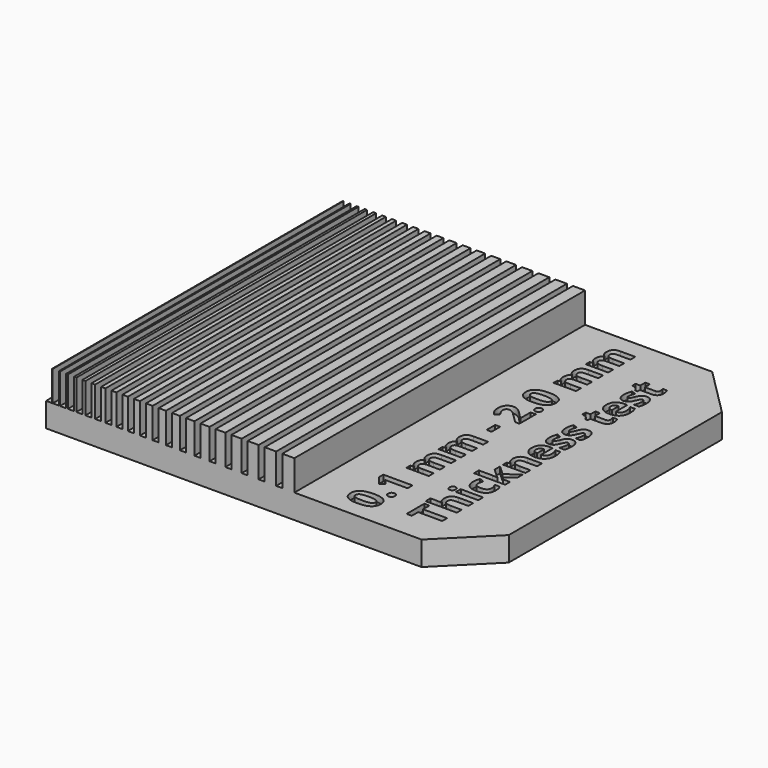
from build123d import *

# Parameters (mm, degrees)
F0_W         = 70
F0_H         = 60
F1_DEPTH     = 4
F2_W         = 0.1
F2_H         = 60
F2_W_2       = 0.2
F2_W_3       = 0.3
F2_W_4       = 0.4
F2_W_5       = 0.5
F2_W_6       = 0.6
F2_W_7       = 0.7
F2_W_8       = 0.8
F2_W_9       = 0.9
F2_W_10      = 1
F2_W_11      = 1.1
F2_W_12      = 1.2
F2_W_13      = 1.3
F2_W_14      = 1.4
F2_W_15      = 1.5
F2_W_16      = 1.6
F2_W_17      = 1.7
F2_W_18      = 1.9
F2_W_19      = 2
F2_W_20      = 1.8
F3_DEPTH     = 5
F4_TEXT_SIZE = 6.7632478961
F5_DEPTH     = 1
F6_SIZE      = 8


# Not quite as in the source:
# - Text() gives the source's letters only with a copy of the font that has no kerning and outlines rounded to 1/6400 em; it was checked with that copy


with BuildPart() as f1:
    # F0 (on Top) → F1 (new body)
    with BuildSketch(Plane.XY):
        Rectangle(F0_W, F0_H)
    extrude(amount=F1_DEPTH)

    # F2 (on face) → F3 (join)
    with BuildSketch(Plane.XY.offset(4)):
        with Locations((-33.95, 0)):
            Rectangle(F2_W, F2_H)
        with Locations((-32.8, 0)):
            Rectangle(F2_W_2, F2_H)
        with Locations((-31.55, 0)):
            Rectangle(F2_W_3, F2_H)
        with Locations((-30.2, 0)):
            Rectangle(F2_W_4, F2_H)
        with Locations((-28.75, 0)):
            Rectangle(F2_W_5, F2_H)
        with Locations((-27.2, 0)):
            Rectangle(F2_W_6, F2_H)
        with Locations((-25.55, 0)):
            Rectangle(F2_W_7, F2_H)
        with Locations((-23.8, 0)):
            Rectangle(F2_W_8, F2_H)
        with Locations((-21.95, 0)):
            Rectangle(F2_W_9, F2_H)
        with Locations((-20, 0)):
            Rectangle(F2_W_10, F2_H)
        with Locations((-17.95, 0)):
            Rectangle(F2_W_11, F2_H)
        with Locations((-15.8, 0)):
            Rectangle(F2_W_12, F2_H)
        with Locations((-13.55, 0)):
            Rectangle(F2_W_13, F2_H)
        with Locations((-11.2, 0)):
            Rectangle(F2_W_14, F2_H)
        with Locations((-8.75, 0)):
            Rectangle(F2_W_15, F2_H)
        with Locations((-6.2, 0)):
            Rectangle(F2_W_16, F2_H)
        with Locations((-3.55, 0)):
            Rectangle(F2_W_17, F2_H)
        with Locations((2.05, 0)):
            Rectangle(F2_W_18, F2_H)
        with Locations((5, 0)):
            Rectangle(F2_W_19, F2_H)
        with Locations((-0.8, 0)):
            Rectangle(F2_W_20, F2_H)
    extrude(amount=F3_DEPTH)

    # F4 (on face) → F5 (cut)
    with BuildSketch(Plane.XY.offset(4)):
        with Locations(Location((16.6463407394, -27.5), (0, 0, 90))):
            Text('0.1 mm - 2.0 mm', F4_TEXT_SIZE, font='Open Sans', font_style=FontStyle.BOLD, text_align=(TextAlign.LEFT, TextAlign.BOTTOM))
        with Locations(Location((25.8443578781, -25.7426123045), (0, 0, 90))):
            Text('Thickness test', F4_TEXT_SIZE, font='Open Sans', font_style=FontStyle.BOLD, text_align=(TextAlign.LEFT, TextAlign.BOTTOM))
    extrude(amount=-F5_DEPTH, mode=Mode.SUBTRACT)

    # F6
    f6_edges = [f1.edges().sort_by_distance(p)[0] for p in [
        (35, -30, 2),
        (35, 30, 2),
    ]]
    chamfer(f6_edges, length=F6_SIZE)


solid = f1.part
